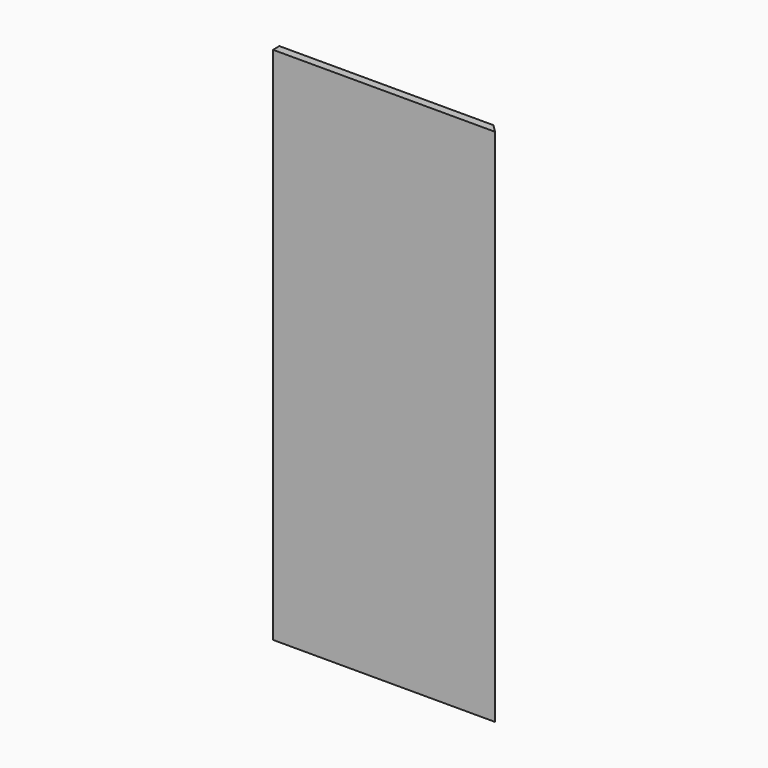
from build123d import *

# Parameters (mm, degrees)
F1_DEPTH = 18
F2_SIZE  = 17.99999


# Not quite as in the source:
# - a fillet or chamfer is up to 0.001 mm smaller than in the source, because OpenCascade refuses the exact size


with BuildPart() as f1:
    # F0 (on Front) → F1 (new body)
    with BuildSketch(Plane.XZ):
        Polygon((0, 0), (-250, 585), (-250, -585), align=None)
        Polygon((250, 585), (-250, 585), (0, 0), align=None)
        Polygon((250, -585), (250, 585), (0, 0), align=None)
        Polygon((0, 0), (-250, -585), (250, -585), align=None)
    extrude(amount=F1_DEPTH)

    # F2 (size 18 in the source; OpenCascade refuses exactly that, so slightly less here)
    f2_edges = [f1.edges().sort_by_distance(p)[0] for p in [
        (250, 0, 0),
    ]]
    chamfer(f2_edges, length=F2_SIZE)


solid = f1.part
